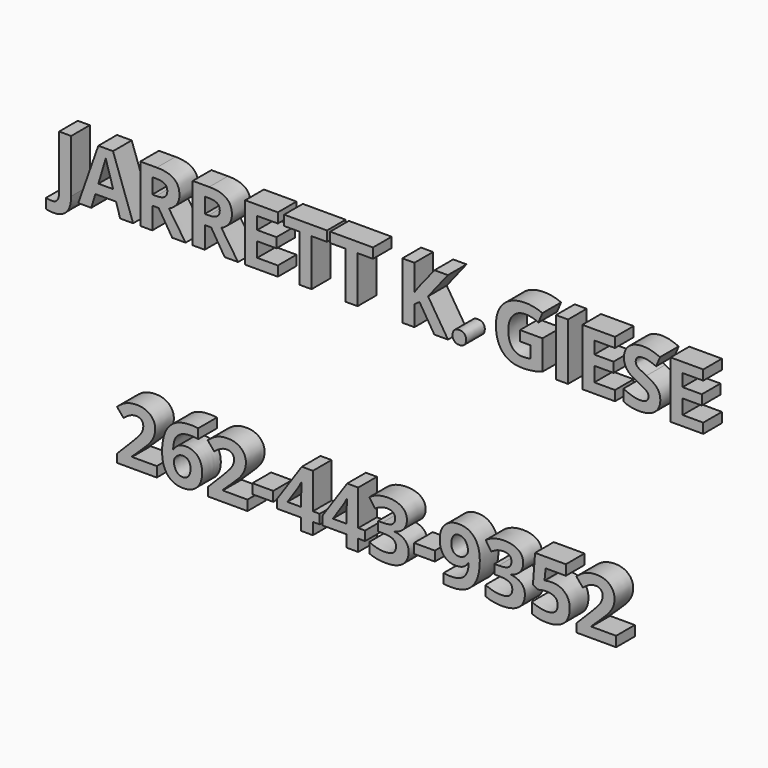
from build123d import *

# Parameters (mm, degrees)
F0_TEXT_SIZE = 86.4714435819
F1_DEPTH     = 25.4


# Not quite as in the source:
# - Text() gives the source's letters only with a copy of the font that has no kerning and outlines rounded to 1/6400 em; it was checked with that copy


with BuildPart() as f1:
    # F0 (on Front) → F1 (new body)
    with BuildSketch(Plane.XZ):
        with Locations((-330.5355012417, 0)):
            Text('JARRETT K. GIESE', F0_TEXT_SIZE, font='Open Sans', font_style=FontStyle.BOLD, text_align=(TextAlign.LEFT, TextAlign.BOTTOM))
        with Locations((-263.128308737, -235.2023265428)):
            Text('262-443-9352', F0_TEXT_SIZE, font='Open Sans', font_style=FontStyle.BOLD, text_align=(TextAlign.LEFT, TextAlign.BOTTOM))
    extrude(amount=F1_DEPTH)


solid = f1.part
